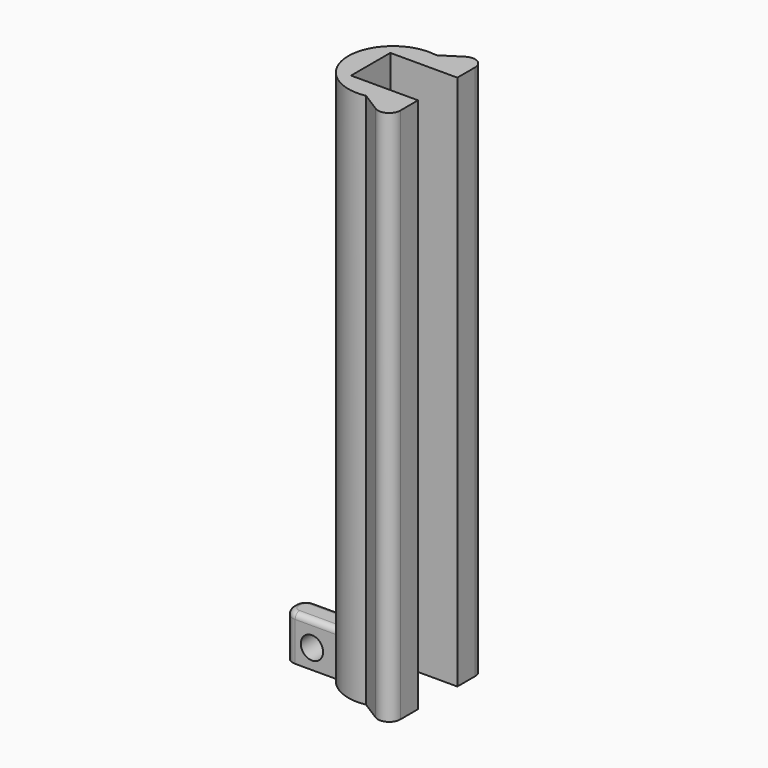
from build123d import *

# Parameters (mm, degrees)
F1_DEPTH = 152.4
F2_DEPTH = 12.7
F3_R     = 3.175
F4_R     = 1.5875
F5_R     = 3.175
F6_DEPTH = 25.4


# Not quite as in the source:
# - a feature names something its author has since deleted; it is built from what else it names


with BuildPart() as f1:
    # F0 (on Top) → F1 (new body)
    with BuildSketch(Plane.XY):
        with BuildLine():
            Line((-6.35, 6.985), (10.6065911112, 6.985))
            ThreePointArc((10.6065911112, 6.985), (7.0295838714, 10.5770955652), (2.33256194, 12.4839558953))
            Line((2.33256194, 12.4839558953), (-6.35, 6.985))
        make_face()
        with BuildLine():
            ThreePointArc((2.33256194, 12.4839558953), (7.0295838714, 10.5770955652), (10.6065911112, 6.985))
            Line((10.6065911112, 6.985), (12.7, 6.985))
            Line((12.7, 6.985), (12.7, 13.2809655419))
            ThreePointArc((12.7, 13.2809655419), (11.0558438219, 16.0625374343), (7.8262096422, 15.9632661068))
            Line((7.8262096422, 15.9632661068), (2.33256194, 12.4839558953))
        make_face()
        with BuildLine():
            Line((12.7, -6.985), (10.6065911112, -6.985))
            ThreePointArc((10.6065911112, -6.985), (7.0295838714, -10.5770955652), (2.33256194, -12.4839558953))
            Line((2.33256194, -12.4839558953), (7.8262096422, -15.9632661068))
            ThreePointArc((7.8262096422, -15.9632661068), (11.0558438219, -16.0625374343), (12.7, -13.2809655419))
            Line((12.7, -13.2809655419), (12.7, -6.985))
        make_face()
        with BuildLine():
            ThreePointArc((2.33256194, -12.4839558953), (7.0295838714, -10.5770955652), (10.6065911112, -6.985))
            Line((10.6065911112, -6.985), (0, -6.985))
            Line((0, -6.985), (-6.35, -6.985))
            Line((-6.35, -6.985), (2.33256194, -12.4839558953))
        make_face()
        with BuildLine():
            Line((-6.35, 6.985), (2.33256194, 12.4839558953))
            ThreePointArc((2.33256194, 12.4839558953), (-8.1137680323, 9.7701979672), (-12.7, 0))
            Line((-12.7, 0), (-6.35, 0))
            Line((-6.35, 0), (-6.35, 6.985))
        make_face()
        with BuildLine():
            ThreePointArc((-10.6065911112, -6.985), (-4.9673452332, -11.6882625456), (2.33256194, -12.4839558953))
            Line((2.33256194, -12.4839558953), (-6.35, -6.985))
            Line((-6.35, -6.985), (-10.6065911112, -6.985))
        make_face()
        with BuildLine():
            Line((-6.35, 0), (-12.7, 0))
            ThreePointArc((-12.7, 0), (-12.1653957419, -3.6459767476), (-10.6065911112, -6.985))
            Line((-10.6065911112, -6.985), (-6.35, -6.985))
            Line((-6.35, -6.985), (-6.35, 0))
        make_face()
    extrude(amount=F1_DEPTH)

    # F0 (on Top) → F2 (join)
    with BuildSketch(Plane.XY):
        with BuildLine():
            Line((-6.35, 0), (-12.7, 0))
            ThreePointArc((-12.7, 0), (-12.1653957419, -3.6459767476), (-10.6065911112, -6.985))
            Line((-10.6065911112, -6.985), (-6.35, -6.985))
            Line((-6.35, -6.985), (-6.35, 0))
        make_face()
        with BuildLine():
            Line((-6.35, 6.985), (2.33256194, 12.4839558953))
            ThreePointArc((2.33256194, 12.4839558953), (-8.1137680323, 9.7701979672), (-12.7, 0))
            Line((-12.7, 0), (-6.35, 0))
            Line((-6.35, 0), (-6.35, 6.985))
        make_face()
        with BuildLine():
            ThreePointArc((-10.6065911112, -6.985), (-12.1653957419, -3.6459767476), (-12.7, 0))
            Line((-12.7, 0), (-25.4, 0))
            Line((-25.4, 0), (-25.4, -6.985))
            Line((-25.4, -6.985), (-10.6065911112, -6.985))
        make_face()
    extrude(amount=F2_DEPTH)

    # F3
    f3_edges = [f1.edges().sort_by_distance(p)[0] for p in [
        (-25.4, 0, 6.35),
        (-25.4, -6.985, 6.35),
    ]]
    fillet(f3_edges, radius=F3_R)

    # F4
    f4_edges = [f1.edges().sort_by_distance(p)[0] for p in [
        (-17.4625, 0, 12.7),
        (-24.470064, -0.929936, 12.7),
        (-25.4, -3.4925, 12.7),
        (-24.470064, -6.055064, 12.7),
        (-16.415796, -6.985, 12.7),
    ]]
    fillet(f4_edges, radius=F4_R)

    # F5 (on face) → F6 (cut)
    with BuildSketch(Plane(origin=(0, 0, 0), x_dir=(-1, 0, 0), z_dir=(0, 1, 0))):
        with Locations((17.4625, 5.55625)):
            Circle(F5_R)
    extrude(amount=-F6_DEPTH, mode=Mode.SUBTRACT)


solid = f1.part
